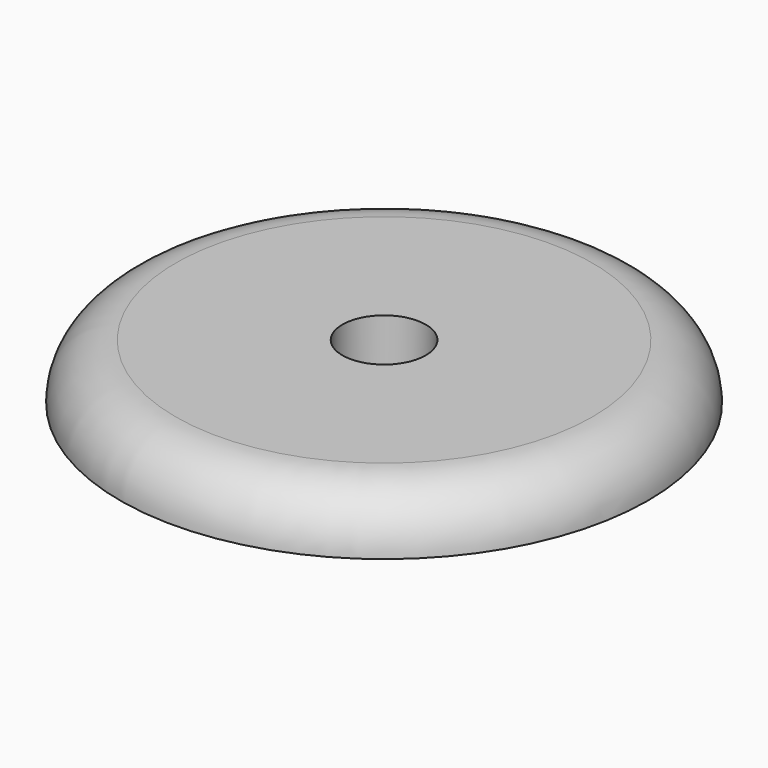
from build123d import *

# Parameters (mm, degrees)
F0_R     = 9.5
F0_R_2   = 1.5
F1_DEPTH = 2
F2_R     = 1.99999


# Not quite as in the source:
# - a fillet or chamfer is up to 0.001 mm smaller than in the source, because OpenCascade refuses the exact size


with BuildPart() as f1:
    # F0 (on Top) → F1 (new body)
    with BuildSketch(Plane.XY):
        Circle(F0_R)
        Circle(F0_R_2, mode=Mode.SUBTRACT)
    extrude(amount=F1_DEPTH)

    # F2 (radius 2 in the source; OpenCascade refuses exactly that, so slightly less here)
    f2_edges = [f1.edges().sort_by_distance(p)[0] for p in [
        (-9.5, 0, 2),
    ]]
    fillet(f2_edges, radius=F2_R)


solid = f1.part
